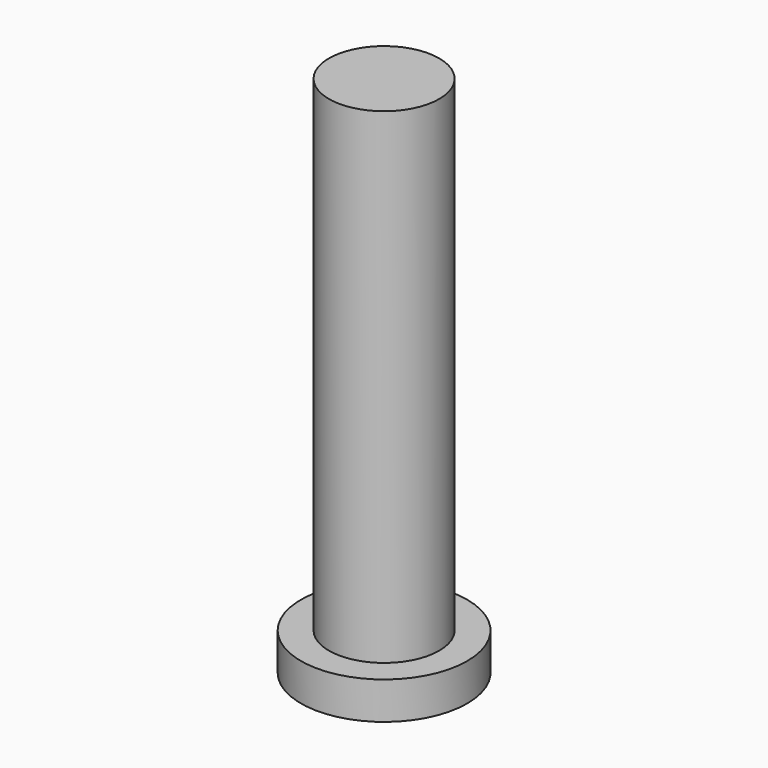
from build123d import *

# Parameters (mm, degrees)
F0_R     = 1.475
F1_DEPTH = 13
F2_R     = 2.225
F2_R_2   = 1.475
F3_DEPTH = 1


with BuildPart() as f1:
    # F0 (on Top) → F1 (new body)
    with BuildSketch(Plane.XY):
        Circle(F0_R)
    extrude(amount=F1_DEPTH)

    # F2 (on face) → F3 (join)
    with BuildSketch(Plane(origin=(0, 0, 0), x_dir=(1, 0, 0), z_dir=(0, 0, -1))):
        Circle(F2_R)
        Circle(F2_R_2, mode=Mode.SUBTRACT)
        Circle(F2_R_2)
    extrude(amount=F3_DEPTH)


solid = f1.part
